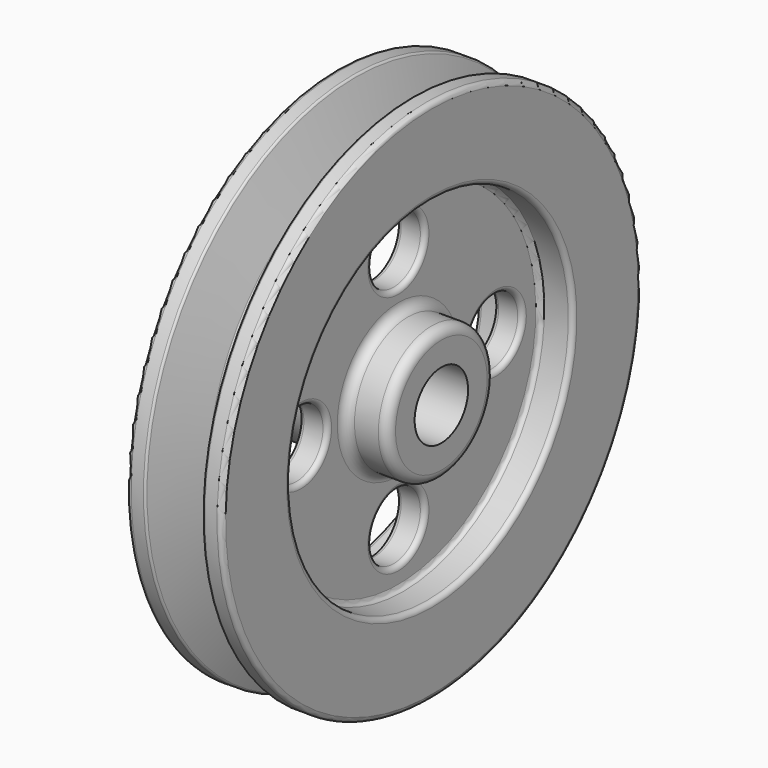
from build123d import *

# Parameters (mm, degrees)
F2_R            = 7
F3_DEPTH        = 6
F3_COPIES_COUNT = 4
F4_R            = 2.5
F5_DEPTH        = 55.0010001
F6_SIZE         = 1
F7_R            = 1


# Not quite as in the source:
# - a pattern or mirror of a feature is missing from the dataset's text; its kind, count and spacing are read off the source's solid


with BuildPart() as f1:
    # F0 (on Front) → F1 (revolve)
    with BuildSketch(Plane.XZ):
        with BuildLine():
            Line((-37, 7), (0, 7))
            Line((0, 7), (0, 12))
            ThreePointArc((0, 12), (-0.5857864376, 13.4142135624), (-2, 14))
            Line((-2, 14), (-7, 14))
            ThreePointArc((-7, 14), (-8.4142135624, 14.5857864376), (-9, 16))
            Line((-9, 16), (-9, 37))
            Line((-9, 37), (-2, 37))
            Line((-2, 37), (-2, 55))
            Line((-2, 55), (-5.5745901029, 55))
            ThreePointArc((-5.5745901029, 55), (-5.8684827291, 54.9045084972), (-6.0501183611, 54.6545084972))
            Line((-6.0501183611, 54.6545084972), (-9.9993575699, 42.5))
            Line((-9.9993575699, 42.5), (-14.0006424301, 42.5))
            Line((-14.0006424301, 42.5), (-17.9498816389, 54.6545084972))
            ThreePointArc((-17.9498816389, 54.6545084972), (-18.1315172709, 54.9045084972), (-18.4254098971, 55))
            Line((-18.4254098971, 55), (-22, 55))
            Line((-22, 55), (-22, 37))
            Line((-22, 37), (-15, 37))
            Line((-15, 37), (-15, 14))
            Line((-15, 14), (-37, 14))
            Line((-37, 14), (-37, 7))
        make_face()
    revolve(axis=Axis((-17.3296256442, 0, 0), (-1, 0, 0)))

    # F2 (on face) → F3 (cut, through all)
    with BuildSketch(Plane(origin=(-15, 0, 0), x_dir=(0, -1, 0), z_dir=(-1, 0, 0))):
        with Locations((0, 25.5)):
            Circle(F2_R)
    f3 = extrude(amount=-F3_DEPTH, mode=Mode.SUBTRACT)

    # F3_copies: F3 ×4 about axis
    f3_copies_axis = Axis((0, 0, 0), (1, 0, 0))
    for i in range(1, F3_COPIES_COUNT):
        add(f3.rotate(f3_copies_axis, i * 360 / F3_COPIES_COUNT), mode=Mode.SUBTRACT)

    # F4 (on Top) → F5 (cut, through all)
    with BuildSketch(Plane.XY):
        with Locations((-29, 0)):
            Circle(F4_R)
    extrude(amount=F5_DEPTH, mode=Mode.SUBTRACT)

    # F6
    f6_edges = [f1.edges().sort_by_distance(p)[0] for p in [
        (-37, 0, -7),
    ]]
    chamfer(f6_edges, length=F6_SIZE)

    # F7
    f7_edges = [f1.edges().sort_by_distance(p)[0] for p in [
        (-37, 0, -14),
        (-15, 0, -37),
        (-22, 0, -37),
        (-22, 0, -55),
        (-15, 0, -14),
        (-15, 7, 25.5),
        (-2, 0, -55),
        (-2, 0, -37),
        (-9, 0, -37),
        (-9, 7, 25.5),
        (-14.000642, 0, -42.5),
        (-9.999358, 0, -42.5),
        (-15, -25.5, 7),
        (-15, -7, -25.5),
        (-15, 25.5, -7),
        (-9, -25.5, 7),
        (-9, -7, -25.5),
        (-9, 25.5, -7),
    ]]
    fillet(f7_edges, radius=F7_R)


solid = f1.part
